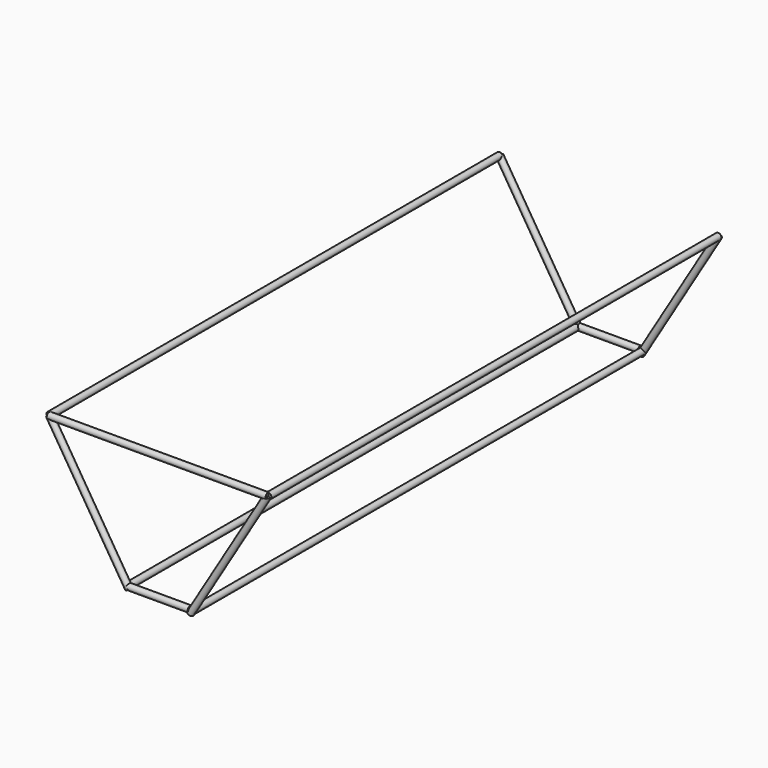
from build123d import *

# Parameters (mm, degrees)
F0_R      = 10
F1_DEPTH  = 1800
F2_DEPTH  = 1800
F3_DEPTH  = 1800
F4_R      = 10
F5_DEPTH  = 100
F6_DEPTH  = 350
F8_R      = 10.0015842189
F9_DEPTH  = 480
F8_R_2    = 10
F10_ANGLE = -32
F11_ANGLE = 31


# Not quite as in the source:
# - a feature names something its author has since deleted; it is built from what else it names
# - the program builds the solid bodies; features that only make, move or delete a surface that nothing else refers to are left out


with BuildPart() as f1:
    # F0 (on Front) → F1 (new body)
    with BuildSketch(Plane.XZ):
        with Locations((-350, 0)):
            Circle(F0_R)
    extrude(amount=F1_DEPTH)

    # F0 (on Front) → F2 (join)
    with BuildSketch(Plane.XZ):
        with Locations((-350, 0)):
            Circle(F0_R)
    extrude(amount=F2_DEPTH)


with BuildPart() as f1b:
    # F0 (on Front) → F1, piece 2 (new body)
    with BuildSketch(Plane.XZ):
        with Locations((350, 0)):
            Circle(F0_R)
    extrude(amount=F1_DEPTH)

    # F0 (on Front) → F2, piece 2 (join)
    with BuildSketch(Plane.XZ):
        with Locations((350, 0)):
            Circle(F0_R)
    extrude(amount=F2_DEPTH)


with BuildPart() as f1c:
    # F0 (on Front) → F1, piece 3 (new body)
    with BuildSketch(Plane.XZ):
        with Locations((110, -400)):
            Circle(F0_R)
    extrude(amount=F1_DEPTH)

    # F0 (on Front) → F2, piece 3 (join)
    with BuildSketch(Plane.XZ):
        with Locations((110, -400)):
            Circle(F0_R)
    extrude(amount=F2_DEPTH)


with BuildPart() as f1d:
    # F0 (on Front) → F1, piece 4 (new body)
    with BuildSketch(Plane.XZ):
        with Locations((-100, -400)):
            Circle(F0_R)
    extrude(amount=F1_DEPTH)

    # F0 (on Front) → F2, piece 4 (join)
    with BuildSketch(Plane.XZ):
        with Locations((-100, -400)):
            Circle(F0_R)
    extrude(amount=F2_DEPTH)


with BuildPart() as f3:
    # F0 (on Front) → F3 (new body)
    with BuildSketch(Plane.XZ):
        with Locations((-350, 0)):
            Circle(F0_R)
    extrude(amount=F3_DEPTH)


with BuildPart() as f3b:
    # F0 (on Front) → F3, piece 2 (new body)
    with BuildSketch(Plane.XZ):
        with Locations((350, 0)):
            Circle(F0_R)
    extrude(amount=F3_DEPTH)


with BuildPart() as f3c:
    # F0 (on Front) → F3, piece 3 (new body)
    with BuildSketch(Plane.XZ):
        with Locations((110, -400)):
            Circle(F0_R)
    extrude(amount=F3_DEPTH)


with BuildPart() as f3d:
    # F0 (on Front) → F3, piece 4 (new body)
    with BuildSketch(Plane.XZ):
        with Locations((-100, -400)):
            Circle(F0_R)
    extrude(amount=F3_DEPTH)


with BuildPart() as f5:
    # F4 (on Right) → F5 (new body, symmetric)
    with BuildSketch(Plane.YZ):
        with Locations((0, -400.0841677189)):
            Circle(F4_R)
    extrude(amount=F5_DEPTH, both=True)


with BuildPart() as f5b:
    # F4 (on Right) → F5, piece 2 (new body, symmetric)
    with BuildSketch(Plane.YZ):
        with Locations((-1800.1378774643, -400.0841677189)):
            Circle(F4_R)
    extrude(amount=F5_DEPTH, both=True)


with BuildPart() as f6:
    # F4 (on Right) → F6 (new body, symmetric)
    with BuildSketch(Plane.YZ):
        with Locations((-1801.4118671417, 0)):
            Circle(F4_R)
    extrude(amount=F6_DEPTH, both=True)


with BuildPart() as f9:
    # F8 (on Top) → F9 (new body)
    with BuildSketch(Plane.XY):
        with Locations((-349.4869470596, -1800.0373840332)):
            Circle(F8_R)
    extrude(amount=-F9_DEPTH)


with BuildPart() as f9b:
    # F8 (on Top) → F9, piece 2 (new body)
    with BuildSketch(Plane.XY):
        with Locations((348.4772145748, -1799.9181747437)):
            Circle(F8_R_2)
    extrude(amount=-F9_DEPTH)


with BuildPart() as f9c:
    # F8 (on Top) → F9, piece 3 (new body)
    with BuildSketch(Plane.XY):
        with Locations((350.0000238419, 0)):
            Circle(F8_R_2)
    extrude(amount=-F9_DEPTH)


with BuildPart() as f9d:
    # F8 (on Top) → F9, piece 4 (new body)
    with BuildSketch(Plane.XY):
        with Locations((-349.9954044819, 0)):
            Circle(F8_R_2)
    extrude(amount=-F9_DEPTH)


with BuildPart() as f9_1:
    # F10: moved
    add(f9.part.rotate(Axis((-350, 0, 0), (0, 1, 0)), F10_ANGLE))


with BuildPart() as f9d_1:
    # F10: moved
    add(f9d.part.rotate(Axis((-350, 0, 0), (0, 1, 0)), F10_ANGLE))


with BuildPart() as f9b_1:
    # F11: moved
    add(f9b.part.rotate(Axis((350, 0, 0), (0, 1, 0)), F11_ANGLE))


with BuildPart() as f9c_1:
    # F11: moved
    add(f9c.part.rotate(Axis((350, 0, 0), (0, 1, 0)), F11_ANGLE))


solid = Compound([f1.part, f1b.part, f1c.part, f1d.part, f3.part, f3b.part, f3c.part, f3d.part, f5.part, f5b.part, f6.part, f9_1.part, f9d_1.part, f9b_1.part, f9c_1.part])
